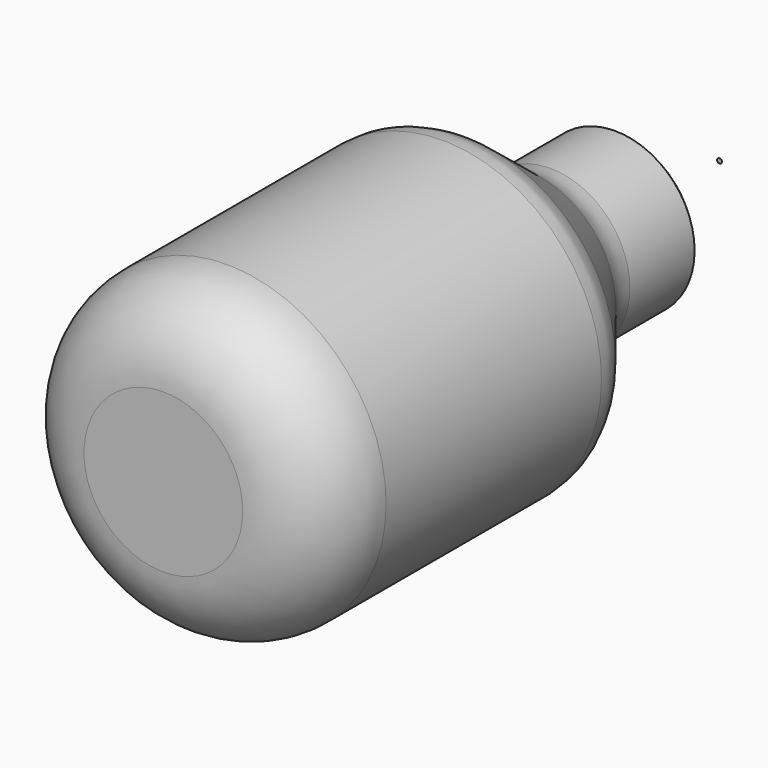
from build123d import *

# Parameters (mm, degrees)
F5_R     = 18.5365010698
F6_DEPTH = 114.3


# Not quite as in the source:
# - a fillet or chamfer that OpenCascade refuses, or shapes differently, is made with other operations: its cross-section is extruded or revolved along the edge and cut away or added


with BuildPart() as f1:
    # F0 (on Top) → F1 (revolve)
    with BuildSketch(Plane.XY):
        with BuildLine():
            Line((0, 84.0317292744), (0, 84.0408968434))
            Line((0, 84.0408968434), (-0.6141534664, 84.0316613536))
            ThreePointArc((-0.6141534664, 84.0316613536), (-0.3070769866, 84.0339870748), (0, 84.0317292744))
        make_face()
    revolve(axis=Axis((0, 84.0363130589, 0), (0, -1, 0)))


with BuildPart() as f1b:
    # F0 (on Top) → F1, piece 2 (revolve)
    with BuildSketch(Plane.XY):
        with BuildLine():
            Line((0, 63.4599872006), (0, -93.2180002618))
            Line((0, -93.2180002618), (20.2258732946, -93.2180002618))
            ThreePointArc((20.2258732946, -93.2180002618), (34.5942830883, -87.2664100555), (40.5458732946, -72.8980002618))
            Line((40.5458732946, -72.8980002618), (40.5458732946, -4.2690273975))
            ThreePointArc((40.5458732946, -4.2690273975), (39.8365270619, -0.084027728), (37.7877280609, 3.6334737133))
            Line((37.7877280609, 3.6334737133), (23.0273435769, 22.2029869316))
            ThreePointArc((23.0273435769, 22.2029869316), (20.9785445759, 25.9204883728), (20.2691983432, 30.1054880424))
            Line((20.2691983432, 30.1054880424), (20.2691983432, 63.4599872006))
            Line((20.2691983432, 63.4599872006), (0, 63.4599872006))
        make_face()
    revolve(axis=Axis((0, 84.0363130589, 0), (0, -1, 0)))

    # F5 (on face) → F6 (cut)
    with BuildSketch(Plane(origin=(0, 63.4599872006, 0), x_dir=(-1, 0, 0), z_dir=(0, 1, 0))):
        Circle(F5_R)
    extrude(amount=-F6_DEPTH, mode=Mode.SUBTRACT)

    # F7: chamfer of 12.7 on 1 edges, made by hand

    # F7_s1 → F7_t2 (revolve, cut)
    with BuildSketch(Plane.XY):
        Polygon((20.2691983432, 50.7599872006), (7.5691983432, 63.4599872006), (20.2691983432, 63.4599872006), align=None)
    revolve(axis=Axis((0, 63.4599872006, 0), (0, -1, 0)), mode=Mode.SUBTRACT)


with BuildPart() as f3:
    # F2 (on Top) → F3 (revolve)
    with BuildSketch(Plane.XY):
        Polygon((0, 62.8846511245), (0, 21.3541854173), (23.9753127098, 21.3541854173), (8.4013864398, 62.8846511245), align=None)
    revolve(axis=Axis((0, 42.1194182709, 0), (0, -1, 0)))


solid = Compound([f1.part, f1b.part])
